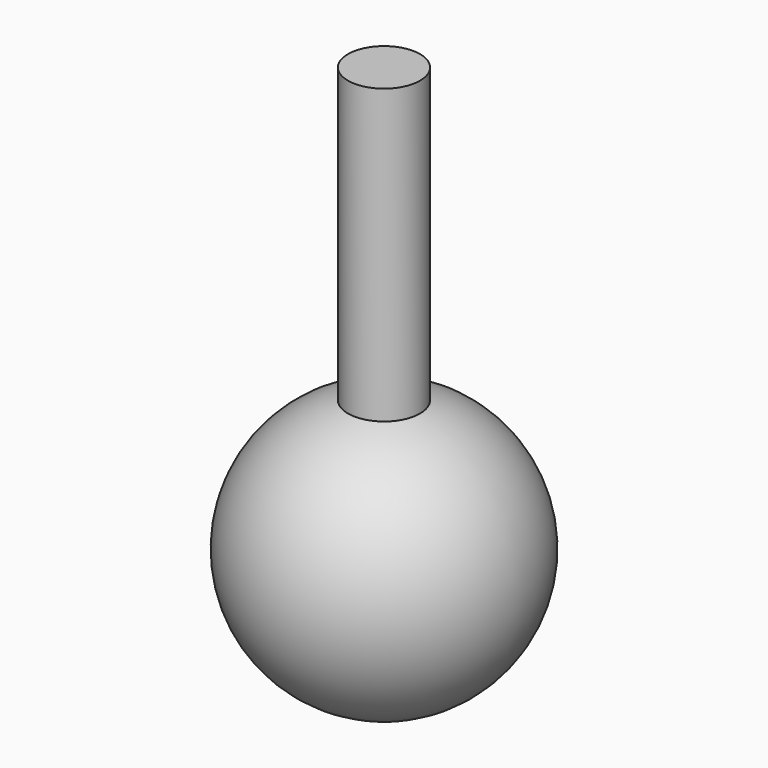
from build123d import *

# Parameters (mm, degrees)
F5_R      = 1.5875
F6_DEPTH  = 12.7
F6_FACE_R = 1.5875


# Not quite as in the source:
# - a variable given as a bare number and used for a length is read in inches; the dataset says mm whatever the document's units were


with BuildPart() as f3:
    # F2 (on Front) → F3 (revolve)
    with BuildSketch(Plane.XZ):
        with BuildLine():
            ThreePointArc((0, -5.969), (5.969, 0), (0, 5.969))
            Line((0, 5.969), (0, -5.969))
        make_face()
    revolve(axis=Axis((0, 0, 0), (0, 0, -1)))

    # F5 (on offset) → F6 (join)
    with BuildSketch(Plane.XY.offset(5.969)):
        Circle(F5_R)
    extrude(amount=F6_DEPTH)

    # F6_face (on face) → F7 (join, up to the next surface of F3)
    with BuildSketch(Plane(origin=(0, 0, 5.969), x_dir=(1, 0, 0), z_dir=(0, 0, -1))):
        Circle(F6_FACE_R)
    extrude(until=Until.NEXT)


solid = f3.part
